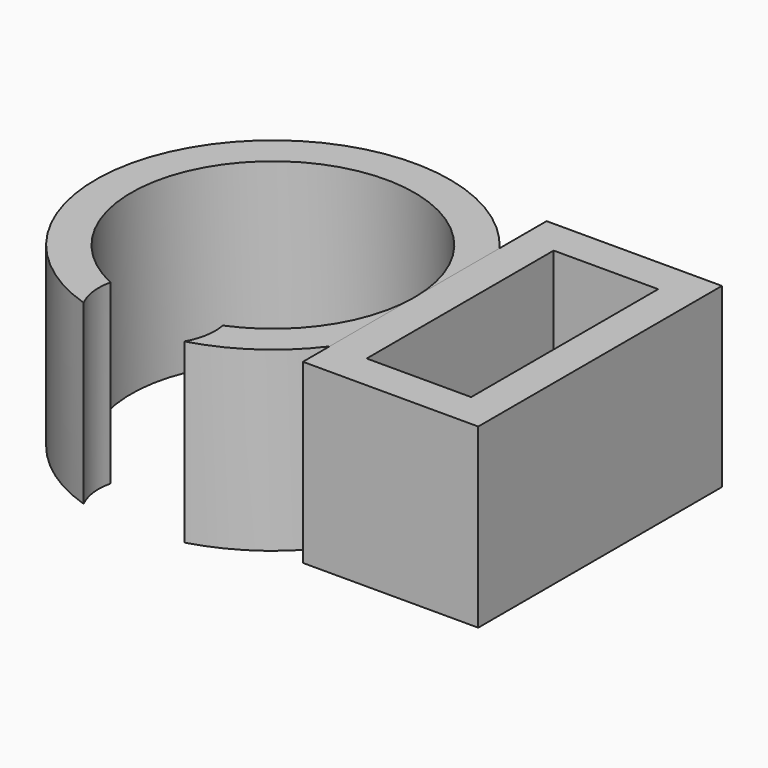
from build123d import *

# Parameters (mm, degrees)
F0_R      = 10
F0_R_2    = 8
F1_DEPTH  = 10
F3_DEPTH  = 10.001
F5_DEPTH  = 10.001
F4_W      = 9.9
F4_H      = 17.2
F6_DEPTH  = 7
F7_W      = 5.9
F7_H      = 13.2
F8_DEPTH  = 25
F9_W      = 9.9
F9_H      = 17.2
F9_W_2    = 2
F9_H_2    = 13.2
F10_DEPTH = 3


# Not quite as in the source:
# - a feature names something its author has since deleted; it is built from what else it names


with BuildPart() as f1:
    # F0 (on Top) → F1 (new body)
    with BuildSketch(Plane.XY):
        with Locations((-52.405577153, 40.0831848383)):
            Circle(F0_R)
        with Locations((-52.405577153, 40.0831848383)):
            Circle(F0_R_2, mode=Mode.SUBTRACT)
    extrude(amount=F1_DEPTH)

    # F2 (on face) → F3 (cut, through all)
    with BuildSketch(Plane.XY.offset(10)):
        with BuildLine():
            ThreePointArc((-49.7031392182, 30.4552655818), (-49.3810314173, 31.2418399469), (-49.2712181951, 32.0846885237))
            ThreePointArc((-49.2712181951, 32.0846885237), (-49.2856908096, 32.3929169306), (-49.3289813029, 32.6984331177))
            ThreePointArc((-49.3289813029, 32.6984331177), (-52.5606793952, 32.0846885237), (-55.7661541698, 32.8232590732))
            ThreePointArc((-55.7661541698, 32.8232590732), (-55.8238565493, 31.6696826825), (-55.4792412657, 30.5672724321))
            ThreePointArc((-55.4792412657, 30.5672724321), (-52.5994549558, 30.0850644451), (-49.7031392182, 30.4552655818))
        make_face()
    extrude(amount=-F3_DEPTH, mode=Mode.SUBTRACT)

    # F4 (on face) → F5 (cut, through all)
    with BuildSketch(Plane.XY.offset(10)):
        with BuildLine():
            ThreePointArc((-44.405577153, 34.0831848383), (-42.405577153, 40.0831848383), (-44.405577153, 46.0831848383))
            Line((-44.405577153, 46.0831848383), (-44.405577153, 40.0831848383))
            Line((-44.405577153, 40.0831848383), (-44.405577153, 34.0831848383))
        make_face()
    extrude(amount=-F5_DEPTH, mode=Mode.SUBTRACT)


with BuildPart() as f6:
    # F4 (on face) → F6 (new body)
    with BuildSketch(Plane.XY.offset(10)):
        with Locations((-39.455577153, 40.8040919366)):
            Rectangle(F4_W, F4_H)
    extrude(amount=-F6_DEPTH)

    # F7 (on face) → F8 (cut)
    with BuildSketch(Plane.XY.offset(10)):
        with Locations((-39.455577153, 40.8040919366)):
            Rectangle(F7_W, F7_H)
    extrude(amount=-F8_DEPTH, mode=Mode.SUBTRACT)

    # F9 (on face) → F10 (join)
    with BuildSketch(Plane(origin=(0, 0, 3), x_dir=(1, 0, 0), z_dir=(0, 0, -1))):
        with Locations((-39.455577153, -40.8040919366)):
            Rectangle(F9_W, F9_H)
        Polygon((-42.405577153, -47.4040919366), (-42.405577153, -34.2040919366), (-40.405577153, -34.2040919366), (-38.505577153, -34.2040919366), (-36.505577153, -34.2040919366), (-36.505577153, -47.4040919366), (-38.505577153, -47.4040919366), (-40.405577153, -47.4040919366), align=None, mode=Mode.SUBTRACT)
        with Locations((-41.405577153, -40.8040919366)):
            Rectangle(F9_W_2, F9_H_2)
        with Locations((-37.505577153, -40.8040919366)):
            Rectangle(F9_W_2, F9_H_2)
    extrude(amount=F10_DEPTH)


solid = Compound([f1.part, f6.part])
